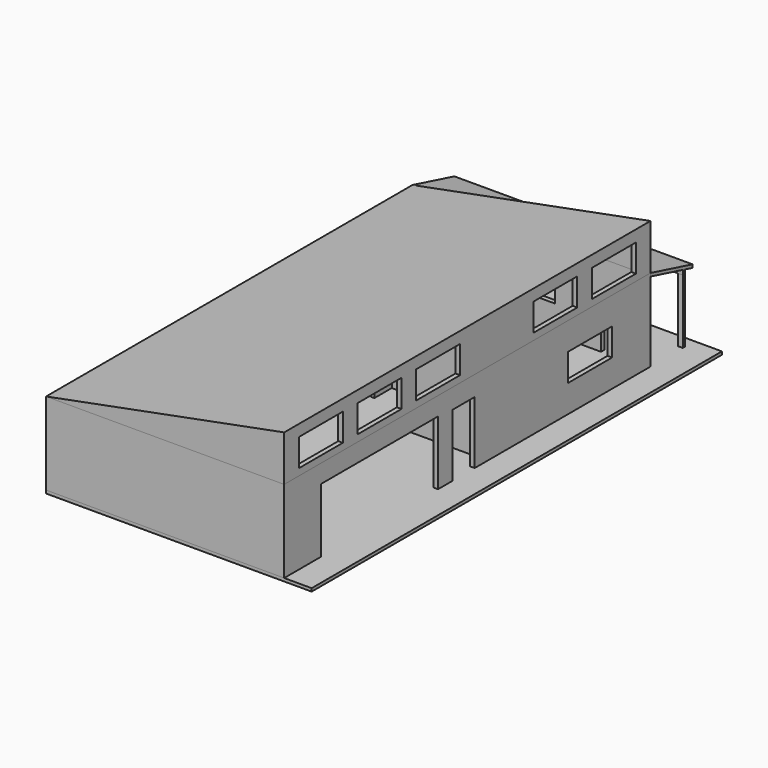
from build123d import *

# Parameters (mm, degrees)
F1_W      = 8839.2
F1_H      = 17068.8
F2_DEPTH  = 101.6
F0_W      = 7924.8
F0_H      = 15240
F0_W_2    = 7620
F0_H_2    = 14935.2
F3_DEPTH  = 2743.2
F5_DEPTH  = 15240
F6_W      = 4876.8
F6_H      = 2133.6
F7_DEPTH  = 304.8
F9_DEPTH  = 7924.8
F10_W     = 609.6
F10_H     = 1524
F10_W_2   = 1828.8
F10_H_2   = 914.4
F10_W_3   = 914.4
F10_H_3   = 2032
F11_DEPTH = 304.8
F12_T     = -152.4
F13_W     = 1828.8
F13_H     = 914.4
F14_DEPTH = 304.8
F15_W     = 101.6
F15_H     = 152.4
F16_DEPTH = 7924.8
F17_W     = 152.4
F17_H     = 101.6
F18_DEPTH = 2209.8
F19_W     = 1524
F19_H     = 1524
F20_DEPTH = 4267.2
F21_W     = 762
F21_H     = 2082.8
F22_DEPTH = 152.4
F23_W     = 762
F23_H     = 2082.8
F23_W_2   = 914.4
F24_DEPTH = 152.4
F25_W     = 1828.8
F25_H     = 914.4
F26_DEPTH = 152.4
F28_DEPTH = 1811.79238
F29_W     = 914.4
F29_H     = 2082.8
F30_DEPTH = 152.4
F31_W     = 762
F31_H     = 2082.8
F32_DEPTH = 152.4


# Not quite as in the source:
# - a feature names something its author has since deleted; it is built from what else it names


with BuildPart() as f2:
    # F1 (on Top) → F2 (new body)
    with BuildSketch(Plane.XY):
        with Locations((4419.6, 8534.4)):
            Rectangle(F1_W, F1_H)
    extrude(amount=-F2_DEPTH)


with BuildPart() as f3:
    # F0 (on Top) → F3 (new body)
    with BuildSketch(Plane.XY):
        with Locations((3962.4, 7620)):
            Rectangle(F0_W, F0_H)
        with Locations((3962.4, 7620)):
            Rectangle(F0_W_2, F0_H_2, mode=Mode.SUBTRACT)
    extrude(amount=F3_DEPTH)

    # F6 (on face) → F7 (cut)
    with BuildSketch(Plane.YZ.offset(7924.8)):
        with Locations((3962.4, 1066.8)):
            Rectangle(F6_W, F6_H)
    extrude(amount=-F7_DEPTH, mode=Mode.SUBTRACT)

    # F10 (on face) → F11 (cut)
    with BuildSketch(Plane(origin=(0, 15240, 0), x_dir=(-1, 0, 0), z_dir=(0, 1, 0))):
        with Locations((-6705.6, 762)):
            Rectangle(F10_W, F10_H)
        with Locations((-3962.4, 1371.6)):
            Rectangle(F10_W_2, F10_H_2)
        with Locations((-1371.6, 1016)):
            Rectangle(F10_W_3, F10_H_3)
    extrude(amount=-F11_DEPTH, mode=Mode.SUBTRACT)

    # F25 (on face) → F26 (cut)
    with BuildSketch(Plane.YZ.offset(7924.8)):
        with Locations((12725.4, 1371.6)):
            Rectangle(F25_W, F25_H)
    extrude(amount=-F26_DEPTH, mode=Mode.SUBTRACT)

    # F29 (on face) → F30 (cut)
    with BuildSketch(Plane.YZ.offset(7924.8)):
        with Locations((7467.6, 1041.4)):
            Rectangle(F29_W, F29_H)
    extrude(amount=-F30_DEPTH, mode=Mode.SUBTRACT)


with BuildPart() as f5:
    # F4 (on face) → F5 (new body)
    with BuildSketch(Plane.XZ):
        Polygon((7924.8, 4267.2), (0, 2743.2), (7924.8, 2743.2), align=None)
    extrude(amount=-F5_DEPTH)

    # F12
    f12_openings = [f5.faces().sort_by_distance(p)[0] for p in [
        (3962.4, 7620, 2743.2),
    ]]
    offset(amount=F12_T, openings=f12_openings)

    # F13 (on face) → F14 (cut)
    with BuildSketch(Plane.YZ.offset(7924.8)):
        with Locations((1524, 3426.6855716705)):
            Rectangle(F13_W, F13_H)
        with Locations((3962.4, 3426.6855716705)):
            Rectangle(F13_W, F13_H)
        with Locations((6400.8, 3426.6855716705)):
            Rectangle(F13_W, F13_H)
        with Locations((11277.6, 3426.6855716705)):
            Rectangle(F13_W, F13_H)
        with Locations((13716, 3426.6855716705)):
            Rectangle(F13_W, F13_H)
    extrude(amount=-F14_DEPTH, mode=Mode.SUBTRACT)


with BuildPart() as f9:
    # F8 (on face) → F9 (new body)
    with BuildSketch(Plane.YZ.offset(7924.8)):
        Polygon((16988.6724450765, 2286), (15240, 2743.2), (15240, 2638.1847650622), (16988.6724450765, 2180.9847650622), align=None)
    extrude(amount=-F9_DEPTH)


with BuildPart() as f16:
    # F15 (on face) → F16 (new body)
    with BuildSketch(Plane.YZ.offset(7924.8)):
        with Locations((16633.0724450765, 2211.0402736471)):
            Rectangle(F15_W, F15_H)
    extrude(amount=-F16_DEPTH)


with BuildPart() as f18:
    # F17 (on face) → F18 (new body)
    with BuildSketch(Plane(origin=(0, 0, 2134.8402736471), x_dir=(1, 0, 0), z_dir=(0, 0, -1))):
        with Locations((7848.6, -16633.0724450765)):
            Rectangle(F17_W, F17_H)
    extrude(amount=F18_DEPTH)


with BuildPart() as f18b:
    # F17 (on face) → F18, piece 2 (new body)
    with BuildSketch(Plane(origin=(0, 0, 2134.8402736471), x_dir=(1, 0, 0), z_dir=(0, 0, -1))):
        with Locations((5257.8, -16633.0724450765)):
            Rectangle(F17_W, F17_H)
    extrude(amount=F18_DEPTH)


with BuildPart() as f18c:
    # F17 (on face) → F18, piece 3 (new body)
    with BuildSketch(Plane(origin=(0, 0, 2134.8402736471), x_dir=(1, 0, 0), z_dir=(0, 0, -1))):
        with Locations((2667, -16633.0724450765)):
            Rectangle(F17_W, F17_H)
    extrude(amount=F18_DEPTH)


with BuildPart() as f18d:
    # F17 (on face) → F18, piece 4 (new body)
    with BuildSketch(Plane(origin=(0, 0, 2134.8402736471), x_dir=(1, 0, 0), z_dir=(0, 0, -1))):
        with Locations((76.2, -16633.0724450765)):
            Rectangle(F17_W, F17_H)
    extrude(amount=F18_DEPTH)


with BuildPart() as f20:
    # F19 (on Top) → F20 (new body)
    with BuildSketch(Plane.XY):
        Polygon((7772.4, 10210.8), (152.4, 10210.8), (152.4, 10096.5), (1676.4, 10096.5), (1676.4, 9601.2), (152.4, 9601.2), (152.4, 9486.9), (1676.4, 9486.9), (1676.4, 8572.5), (152.4, 8572.5), (152.4, 8458.2), (3429, 8458.2), (3429, 10096.5), (4953, 10096.5), (4953, 8458.2), (7772.4, 8458.2), (7772.4, 8572.5), (5067.3, 8572.5), (5067.3, 10096.5), (7772.4, 10096.5), align=None)
        with Locations((2552.7, 9334.5)):
            Rectangle(F19_W, F19_H, mode=Mode.SUBTRACT)
    extrude(amount=F20_DEPTH)

    # F21 (on face) → F22 (cut)
    with BuildSketch(Plane.XZ.offset(-8458.2)):
        with Locations((838.2, 1041.4)):
            Rectangle(F21_W, F21_H)
    extrude(amount=-F22_DEPTH, mode=Mode.SUBTRACT)

    # F23 (on face) → F24 (cut)
    with BuildSketch(Plane(origin=(0, 10210.8, 0), x_dir=(-1, 0, 0), z_dir=(0, 1, 0))):
        with Locations((-838.2, 1041.4)):
            Rectangle(F23_W, F23_H)
        with Locations((-4191, 1041.4)):
            Rectangle(F23_W_2, F23_H)
        with Locations((-5753.1, 1041.4)):
            Rectangle(F23_W, F23_H)
    extrude(amount=-F24_DEPTH, mode=Mode.SUBTRACT)

    # F27 (on face) → F28 (cut)
    with BuildSketch(Plane(origin=(0, 10210.8, 0), x_dir=(-1, 0, 0), z_dir=(0, 1, 0))):
        Polygon((-7772.4, 4267.2), (-7772.4, 4192.5565476095), (-152.4, 2702.1246839401), (-152.4, 4267.2), align=None)
    extrude(amount=-F28_DEPTH, mode=Mode.SUBTRACT)

    # F31 (on face) → F32 (cut)
    with BuildSketch(Plane.YZ.offset(3429)):
        with Locations((8991.6, 1041.4)):
            Rectangle(F31_W, F31_H)
    extrude(amount=-F32_DEPTH, mode=Mode.SUBTRACT)


solid = Compound([f2.part, f3.part, f5.part, f9.part, f16.part, f18.part, f18b.part, f18c.part, f18d.part, f20.part])
